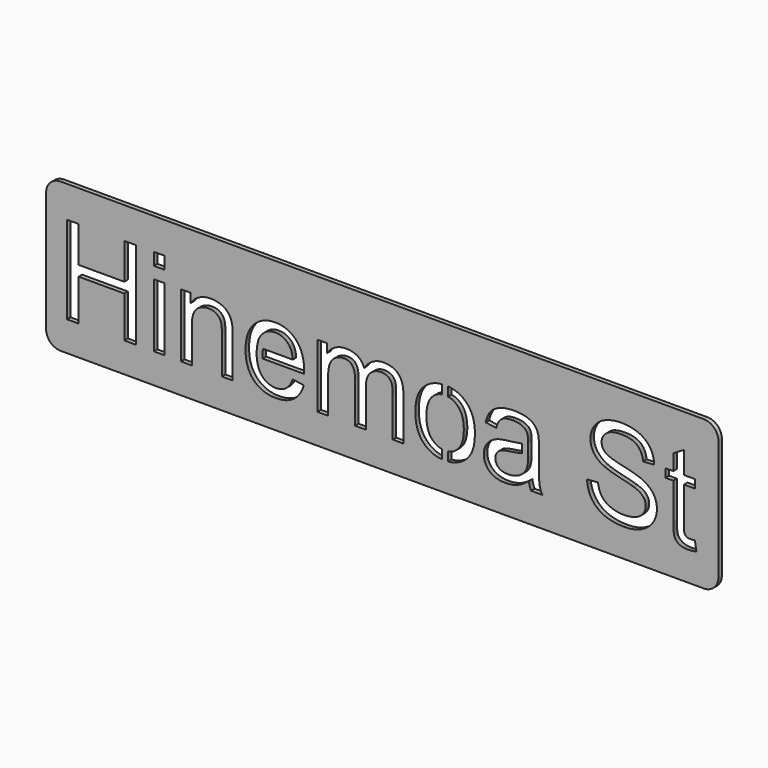
from build123d import *

# Parameters (mm, degrees)
F0_W     = 7.366985
F0_H     = 43.465211
F0_H_2   = 8.472033
F1_DEPTH = 3


# Not quite as in the source:
# - ends of sketch curves that miss each other by under 0.0002 mm in the source are joined


with BuildPart() as f1:
    # F0 (on Front) → F1 (new body)
    with BuildSketch(Plane.XZ):
        with BuildLine():
            Line((-230, 41), (-230, -41))
            ThreePointArc((-230, -41), (-227.0710678119, -48.0710678119), (-220, -51))
            Line((-220, -51), (220, -51))
            ThreePointArc((220, -51), (227.0710678119, -48.0710678119), (230, -41))
            Line((230, -41), (230, 41))
            ThreePointArc((230, 41), (227.0710678119, 48.0710678119), (220, 51))
            Line((220, 51), (-220, 51))
            ThreePointArc((-220, 51), (-227.0710678119, 48.0710678119), (-230, 41))
        make_face()
        Polygon((-207.702338, -2.27893), (-207.702338, -30.559967), (-215.64231, -30.559967), (-215.64231, 29.440033), (-207.702338, 29.440033), (-207.702338, 4.801561), (-176.515435, 4.801561), (-176.515435, 29.440033), (-168.575462, 29.440033), (-168.575462, -30.559967), (-176.515435, -30.559967), (-176.515435, -2.27893), align=None, mode=Mode.SUBTRACT)
        with Locations((-152.5727335, -8.8273615)):
            Rectangle(F0_W, F0_H, mode=Mode.SUBTRACT)
        Polygon((-130.308068, -6.821904), (-130.308068, -30.559967), (-137.675053, -30.559967), (-137.675053, 12.905244), (-131.044766, 12.905244), (-131.044766, 6.725163), (-130.429572, 7.592478), (-129.781124, 8.403837), (-129.099422, 9.159241), (-128.384466, 9.858689), (-127.636257, 10.502181), (-126.854793, 11.089717), (-126.040077, 11.621298), (-125.192106, 12.096922), (-124.310881, 12.516591), (-123.396403, 12.880304), (-122.448671, 13.188061), (-121.467686, 13.439862), (-120.453446, 13.635708), (-119.405953, 13.775597), (-118.325206, 13.859531), (-117.211205, 13.887509), (-116.238853, 13.865446), (-115.286325, 13.799259), (-114.353621, 13.688946), (-113.440742, 13.534508), (-112.547686, 13.335944), (-111.674456, 13.093256), (-110.821049, 12.806442), (-109.987467, 12.475504), (-109.189697, 12.108753), (-108.443726, 11.714504), (-107.749554, 11.292757), (-107.107181, 10.843512), (-106.516607, 10.366768), (-105.977832, 9.862526), (-105.490857, 9.330786), (-105.05568, 8.771547), (-104.661751, 8.18513), (-104.298518, 7.571854), (-103.96598, 6.931719), (-103.664139, 6.264726), (-103.392993, 5.570874), (-103.152542, 4.850163), (-102.942788, 4.102593), (-102.763729, 3.328164), (-102.714168, 3.060375), (-102.667805, 2.768606), (-102.624639, 2.452855), (-102.584671, 2.113123), (-102.5479, 1.74941), (-102.514326, 1.361716), (-102.48395, 0.950041), (-102.456772, 0.514385), (-102.432791, 0.054748), (-102.412007, -0.428871), (-102.394421, -0.93647), (-102.380032, -1.46805), (-102.368841, -2.023612), (-102.360847, -2.603154), (-102.356051, -3.206678), (-102.354452, -3.834183), (-102.354452, -30.559967), (-109.721437, -30.559967), (-109.721437, -4.120677), (-109.734867, -3.030657), (-109.775155, -2.011621), (-109.842302, -1.06357), (-109.936308, -0.186502), (-110.057172, 0.619582), (-110.204896, 1.354682), (-110.379478, 2.018797), (-110.580919, 2.611929), (-110.816573, 3.1555), (-111.093794, 3.670933), (-111.412582, 4.158229), (-111.772938, 4.617386), (-112.174861, 5.048406), (-112.618351, 5.451288), (-113.103408, 5.826032), (-113.630032, 6.172639), (-114.189271, 6.484393), (-114.772171, 6.754579), (-115.378732, 6.983199), (-116.008954, 7.170251), (-116.662838, 7.315736), (-117.340383, 7.419654), (-118.04159, 7.482005), (-118.766458, 7.502789), (-119.349757, 7.491118), (-119.922985, 7.456106), (-120.48614, 7.397752), (-121.039224, 7.316056), (-121.582235, 7.211019), (-122.115175, 7.08264), (-122.638042, 6.93092), (-123.150837, 6.755858), (-123.65356, 6.557455), (-124.146211, 6.33571), (-124.62879, 6.090623), (-125.101298, 5.822195), (-125.563732, 5.530426), (-126.016095, 5.215314), (-126.458386, 4.876861), (-126.890605, 4.515067), (-127.304438, 4.120658), (-127.691573, 3.684363), (-128.052008, 3.20618), (-128.385745, 2.686111), (-128.692783, 2.124154), (-128.973121, 1.520311), (-129.226761, 0.874581), (-129.453702, 0.186963), (-129.653944, -0.542541), (-129.827487, -1.313932), (-129.974331, -2.12721), (-130.094476, -2.982375), (-130.187922, -3.879427), (-130.25467, -4.818366), (-130.294718, -5.799192), align=None, mode=Mode.SUBTRACT)
        with BuildLine():
            ThreePointArc((-81.8910878389, -10.7100350654), (-81.9384658936, -7.6725767513), (-81.6083677497, -4.6527368704))
            Line((-81.6083677497, -4.6527368704), (-61.222119, -4.652737))
            Line((-61.222119, -4.652737), (-61.290545, -3.977909))
            Line((-61.290545, -3.977909), (-61.37304, -3.324505))
            Line((-61.37304, -3.324505), (-61.469604, -2.692524))
            Line((-61.469604, -2.692524), (-61.580237, -2.081966))
            Line((-61.580237, -2.081966), (-61.704938, -1.492831))
            Line((-61.704938, -1.492831), (-61.843709, -0.925119))
            Line((-61.843709, -0.925119), (-61.996548, -0.37883))
            Line((-61.996548, -0.37883), (-62.163456, 0.146036))
            Line((-62.163456, 0.146036), (-62.344434, 0.649478))
            Line((-62.344434, 0.649478), (-62.53948, 1.131498))
            Line((-62.53948, 1.131498), (-62.748595, 1.592094))
            Line((-62.748595, 1.592094), (-62.971778, 2.031268))
            Line((-62.971778, 2.031268), (-63.209031, 2.449018))
            Line((-63.209031, 2.449018), (-63.460353, 2.845345))
            Line((-63.460353, 2.845345), (-63.725743, 3.220249))
            Line((-63.725743, 3.220249), (-64.005203, 3.57373))
            Line((-64.005203, 3.57373), (-64.453329, 4.089163))
            Line((-64.453329, 4.089163), (-64.917762, 4.571343))
            Line((-64.917762, 4.571343), (-65.398503, 5.020268))
            Line((-65.398503, 5.020268), (-65.895551, 5.43594))
            Line((-65.895551, 5.43594), (-66.408905, 5.818358))
            Line((-66.408905, 5.818358), (-66.938567, 6.167523))
            Line((-66.938567, 6.167523), (-67.484536, 6.483433))
            Line((-67.484536, 6.483433), (-68.046813, 6.76609))
            Line((-68.046813, 6.76609), (-68.625396, 7.015493))
            Line((-68.625396, 7.015493), (-69.220286, 7.231643))
            Line((-69.220286, 7.231643), (-69.831484, 7.414538))
            Line((-69.831484, 7.414538), (-70.458989, 7.56418))
            Line((-70.458989, 7.56418), (-71.1028, 7.680568))
            Line((-71.1028, 7.680568), (-71.762919, 7.763703))
            Line((-71.762919, 7.763703), (-72.439345, 7.813583))
            Line((-72.439345, 7.813583), (-73.132079, 7.83021))
            Line((-73.132079, 7.83021), (-73.760143, 7.816941))
            Line((-73.760143, 7.816941), (-74.375577, 7.777132))
            Line((-74.375577, 7.777132), (-74.978381, 7.710785))
            Line((-74.978381, 7.710785), (-75.568555, 7.617898))
            Line((-75.568555, 7.617898), (-76.146099, 7.498472))
            Line((-76.146099, 7.498472), (-76.711014, 7.352507))
            Line((-76.711014, 7.352507), (-77.263298, 7.180003))
            Line((-77.263298, 7.180003), (-77.802952, 6.980961))
            Line((-77.802952, 6.980961), (-78.329976, 6.755379))
            Line((-78.329976, 6.755379), (-78.84437, 6.503258))
            Line((-78.84437, 6.503258), (-79.346134, 6.224598))
            Line((-79.346134, 6.224598), (-79.835267, 5.919399))
            Line((-79.835267, 5.919399), (-80.311771, 5.58766))
            Line((-80.311771, 5.58766), (-80.775645, 5.229383))
            Line((-80.775645, 5.229383), (-81.226889, 4.844567))
            Line((-81.226889, 4.844567), (-81.665503, 4.433212))
            Line((-81.665503, 4.433212), (-82.085731, 3.999634))
            Line((-82.085731, 3.999634), (-82.481818, 3.54815))
            Line((-82.481818, 3.54815), (-82.853765, 3.078761))
            Line((-82.853765, 3.078761), (-83.20157, 2.591465))
            Line((-83.20157, 2.591465), (-83.525235, 2.086264))
            Line((-83.525235, 2.086264), (-83.824758, 1.563157))
            Line((-83.824758, 1.563157), (-84.100141, 1.022144))
            Line((-84.100141, 1.022144), (-84.351383, 0.463225))
            Line((-84.351383, 0.463225), (-84.578484, -0.113599))
            Line((-84.578484, -0.113599), (-84.960261, -1.320966))
            ThreePointArc((-84.960261, -1.320966), (-85.8232752784, -5.9761863774), (-85.901515741, -10.7100800496))
            Line((-85.901515741, -10.7100800496), (-85.87971, -11.011642))
            ThreePointArc((-85.87971, -11.011642), (-85.6041419553, -13.325925097), (-85.1398797958, -15.6098481961))
            Line((-85.1398797958, -15.6098481961), (-84.68392, -17.033364))
            Line((-84.68392, -17.033364), (-84.41805, -17.705793))
            Line((-84.41805, -17.705793), (-84.12692, -18.352003))
            Line((-84.12692, -18.352003), (-83.81053, -18.971994))
            Line((-83.81053, -18.971994), (-83.468879, -19.565765))
            Line((-83.468879, -19.565765), (-83.101969, -20.133317))
            Line((-83.101969, -20.133317), (-82.709799, -20.67465))
            Line((-82.709799, -20.67465), (-82.292368, -21.189763))
            Line((-82.292368, -21.189763), (-81.849677, -21.678657))
            Line((-81.849677, -21.678657), (-81.387322, -22.139574))
            Line((-81.387322, -22.139574), (-80.910898, -22.570753))
            Line((-80.910898, -22.570753), (-80.420406, -22.972196))
            Line((-80.420406, -22.972196), (-79.915844, -23.343903))
            Line((-79.915844, -23.343903), (-79.397213, -23.685873))
            Line((-79.397213, -23.685873), (-78.864514, -23.998107))
            Line((-78.864514, -23.998107), (-78.317745, -24.280604))
            Line((-78.317745, -24.280604), (-77.756908, -24.533364))
            Line((-77.756908, -24.533364), (-77.182002, -24.756388))
            Line((-77.182002, -24.756388), (-76.593027, -24.949675))
            Line((-76.593027, -24.949675), (-75.989983, -25.113226))
            Line((-75.989983, -25.113226), (-75.37287, -25.247041))
            Line((-75.37287, -25.247041), (-74.741688, -25.351119))
            Line((-74.741688, -25.351119), (-74.096437, -25.42546))
            Line((-74.096437, -25.42546), (-73.437118, -25.470065))
            Line((-73.437118, -25.470065), (-72.763729, -25.484933))
            Line((-72.763729, -25.484933), (-71.769314, -25.451679))
            Line((-71.769314, -25.451679), (-70.81199, -25.351918))
            Line((-70.81199, -25.351918), (-69.891756, -25.185649))
            Line((-69.891756, -25.185649), (-69.008613, -24.952873))
            Line((-69.008613, -24.952873), (-68.162561, -24.653589))
            Line((-68.162561, -24.653589), (-67.3536, -24.287798))
            Line((-67.3536, -24.287798), (-66.581729, -23.855499))
            Line((-66.581729, -23.855499), (-65.846949, -23.356693))
            Line((-65.846949, -23.356693), (-65.14926, -22.784984))
            Line((-65.14926, -22.784984), (-64.488661, -22.133978))
            Line((-64.488661, -22.133978), (-63.865153, -21.403674))
            Line((-63.865153, -21.403674), (-63.278736, -20.594074))
            Line((-63.278736, -20.594074), (-62.72941, -19.705175))
            Line((-62.72941, -19.705175), (-62.217174, -18.736979))
            Line((-62.217174, -18.736979), (-61.742029, -17.689486))
            Line((-61.742029, -17.689486), (-61.303975, -16.562696))
            Line((-61.303975, -16.562696), (-53.691424, -17.504033))
            Line((-53.691424, -17.504033), (-53.928517, -18.326264))
            Line((-53.928517, -18.326264), (-54.18959, -19.125153))
            Line((-54.18959, -19.125153), (-54.474645, -19.900701))
            Line((-54.474645, -19.900701), (-54.783682, -20.652907))
            Line((-54.783682, -20.652907), (-55.116699, -21.381772))
            Line((-55.116699, -21.381772), (-55.473697, -22.087295))
            Line((-55.473697, -22.087295), (-55.854676, -22.769476))
            Line((-55.854676, -22.769476), (-56.259637, -23.428316))
            Line((-56.259637, -23.428316), (-56.688578, -24.063815))
            Line((-56.688578, -24.063815), (-57.1415, -24.675972))
            Line((-57.1415, -24.675972), (-57.618404, -25.264787))
            Line((-57.618404, -25.264787), (-58.119289, -25.83026))
            Line((-58.119289, -25.83026), (-58.644154, -26.372392))
            Line((-58.644154, -26.372392), (-59.193001, -26.891183))
            Line((-59.193001, -26.891183), (-59.765829, -27.386632))
            Line((-59.765829, -27.386632), (-60.362638, -27.858739))
            Line((-60.362638, -27.858739), (-60.981989, -28.304787))
            Line((-60.981989, -28.304787), (-61.622443, -28.722058))
            Line((-61.622443, -28.722058), (-62.284001, -29.110551))
            Line((-62.284001, -29.110551), (-62.966662, -29.470267))
            Line((-62.966662, -29.470267), (-63.670427, -29.801206))
            Line((-63.670427, -29.801206), (-64.395295, -30.103367))
            Line((-64.395295, -30.103367), (-65.141266, -30.376752))
            Line((-65.141266, -30.376752), (-65.90834, -30.621359))
            Line((-65.90834, -30.621359), (-66.696518, -30.837188))
            Line((-66.696518, -30.837188), (-67.5058, -31.024241))
            Line((-67.5058, -31.024241), (-68.336184, -31.182516))
            Line((-68.336184, -31.182516), (-69.187672, -31.312013))
            Line((-69.187672, -31.312013), (-70.060263, -31.412734))
            Line((-70.060263, -31.412734), (-70.953958, -31.484677))
            Line((-70.953958, -31.484677), (-71.868756, -31.527843))
            Line((-71.868756, -31.527843), (-72.804657, -31.542232))
            Line((-72.804657, -31.542232), (-73.981248, -31.51929))
            Line((-73.981248, -31.51929), (-75.126984, -31.450464))
            Line((-75.126984, -31.450464), (-76.241864, -31.335755))
            Line((-76.241864, -31.335755), (-77.325888, -31.175161))
            Line((-77.325888, -31.175161), (-78.379057, -30.968684))
            Line((-78.379057, -30.968684), (-79.40137, -30.716324))
            Line((-79.40137, -30.716324), (-80.392827, -30.418079))
            Line((-80.392827, -30.418079), (-81.353429, -30.073951))
            Line((-81.353429, -30.073951), (-82.283175, -29.683939))
            Line((-82.283175, -29.683939), (-83.182066, -29.248043))
            Line((-83.182066, -29.248043), (-84.050101, -28.766263))
            Line((-84.050101, -28.766263), (-84.88728, -28.238599))
            Line((-84.88728, -28.238599), (-85.693603, -27.665052))
            Line((-85.693603, -27.665052), (-86.469071, -27.045621))
            Line((-86.469071, -27.045621), (-87.213683, -26.380306))
            Line((-87.213683, -26.380306), (-87.92744, -25.669108))
            Line((-87.92744, -25.669108), (-88.603946, -24.916502))
            Line((-88.603946, -24.916502), (-89.236807, -24.126965))
            Line((-89.236807, -24.126965), (-89.826021, -23.300497))
            Line((-89.826021, -23.300497), (-90.371591, -22.437099))
            Line((-90.371591, -22.437099), (-90.873515, -21.536769))
            Line((-90.873515, -21.536769), (-91.331793, -20.599509))
            Line((-91.331793, -20.599509), (-91.746426, -19.625318))
            Line((-91.746426, -19.625318), (-92.117413, -18.614196))
            Line((-92.117413, -18.614196), (-92.444754, -17.566144))
            Line((-92.444754, -17.566144), (-92.72845, -16.48116))
            Line((-92.72845, -16.48116), (-92.968501, -15.359246))
            Line((-92.968501, -15.359246), (-93.164906, -14.2004))
            Line((-93.164906, -14.2004), (-93.317665, -13.004624))
            Line((-93.317665, -13.004624), (-93.426779, -11.771917))
            Line((-93.426779, -11.771917), (-93.492248, -10.502279))
            Line((-93.492248, -10.502279), (-93.51407, -9.195711))
            Line((-93.51407, -9.195711), (-93.492008, -7.843818))
            Line((-93.492008, -7.843818), (-93.42582, -6.530295))
            Line((-93.42582, -6.530295), (-93.315507, -5.255141))
            Line((-93.315507, -5.255141), (-93.161069, -4.018357))
            Line((-93.161069, -4.018357), (-92.962506, -2.819943))
            Line((-92.962506, -2.819943), (-92.719817, -1.659899))
            Line((-92.719817, -1.659899), (-92.433004, -0.538224))
            Line((-92.433004, -0.538224), (-92.102065, 0.545081))
            Line((-92.102065, 0.545081), (-91.727001, 1.590016))
            Line((-91.727001, 1.590016), (-91.307812, 2.596581))
            Line((-91.307812, 2.596581), (-90.844498, 3.564777))
            Line((-90.844498, 3.564777), (-90.337058, 4.494603))
            Line((-90.337058, 4.494603), (-89.785493, 5.38606))
            Line((-89.785493, 5.38606), (-89.189804, 6.239146))
            Line((-89.189804, 6.239146), (-88.549989, 7.053863))
            Line((-88.549989, 7.053863), (-87.866049, 7.83021))
            Line((-87.866049, 7.83021), (-87.146936, 8.563711))
            Line((-87.146936, 8.563711), (-86.401604, 9.24989))
            Line((-86.401604, 9.24989), (-85.630053, 9.888745))
            Line((-85.630053, 9.888745), (-84.832283, 10.480278))
            Line((-84.832283, 10.480278), (-84.008294, 11.024489))
            Line((-84.008294, 11.024489), (-83.158085, 11.521377))
            Line((-83.158085, 11.521377), (-82.281656, 11.970942))
            Line((-82.281656, 11.970942), (-81.379009, 12.373184))
            Line((-81.379009, 12.373184), (-80.450142, 12.728104))
            Line((-80.450142, 12.728104), (-79.495056, 13.035701))
            Line((-79.495056, 13.035701), (-78.513751, 13.295976))
            Line((-78.513751, 13.295976), (-77.506226, 13.508928))
            Line((-77.506226, 13.508928), (-76.472482, 13.674557))
            Line((-76.472482, 13.674557), (-75.412519, 13.792864))
            Line((-75.412519, 13.792864), (-74.326336, 13.863848))
            Line((-74.326336, 13.863848), (-73.213934, 13.887509))
            Line((-73.213934, 13.887509), (-72.136704, 13.864327))
            Line((-72.136704, 13.864327), (-71.084415, 13.794782))
            Line((-71.084415, 13.794782), (-70.057066, 13.678874))
            Line((-70.057066, 13.678874), (-69.054657, 13.516602))
            Line((-69.054657, 13.516602), (-68.077189, 13.307966))
            Line((-68.077189, 13.307966), (-67.12466, 13.052968))
            Line((-67.12466, 13.052968), (-66.197073, 12.751606))
            Line((-66.197073, 12.751606), (-65.294425, 12.40388))
            Line((-65.294425, 12.40388), (-64.416718, 12.009791))
            Line((-64.416718, 12.009791), (-63.563951, 11.569339))
            Line((-63.563951, 11.569339), (-62.736124, 11.082523))
            Line((-62.736124, 11.082523), (-61.933238, 10.549344))
            Line((-61.933238, 10.549344), (-61.155292, 9.969801))
            Line((-61.155292, 9.969801), (-60.402287, 9.343895))
            Line((-60.402287, 9.343895), (-59.674221, 8.671626))
            Line((-59.674221, 8.671626), (-58.971096, 7.952993))
            Line((-58.971096, 7.952993), (-58.302024, 7.192314))
            Line((-58.302024, 7.192314), (-57.676118, 6.393904))
            Line((-57.676118, 6.393904), (-57.093378, 5.557764))
            Line((-57.093378, 5.557764), (-56.553804, 4.683894))
            Line((-56.553804, 4.683894), (-56.057396, 3.772293))
            Line((-56.057396, 3.772293), (-55.604154, 2.822963))
            Line((-55.604154, 2.822963), (-55.194078, 1.835902))
            Line((-55.194078, 1.835902), (-54.827167, 0.811111))
            Line((-54.827167, 0.811111), (-54.503423, -0.251411))
            Line((-54.503423, -0.251411), (-54.222844, -1.351662))
            Line((-54.222844, -1.351662), (-53.985432, -2.489644))
            Line((-53.985432, -2.489644), (-53.791185, -3.665356))
            Line((-53.791185, -3.665356), (-53.640104, -4.878798))
            Line((-53.640104, -4.878798), (-53.532189, -6.12997))
            Line((-53.532189, -6.12997), (-53.467441, -7.418873))
            Line((-53.467441, -7.418873), (-53.445858, -8.745506))
            Line((-53.445858, -8.745506), (-53.448416, -9.113855))
            Line((-53.448416, -9.113855), (-53.456089, -9.56406))
            Line((-53.456089, -9.56406), (-53.468879, -10.09612))
            Line((-53.468879, -10.09612), (-53.486785, -10.710035))
            Line((-53.486785, -10.710035), (-81.8910878389, -10.7100350654))
        make_face(mode=Mode.SUBTRACT)
        Polygon((-37.07478, -8.008807), (-37.07478, -30.559967), (-44.441765, -30.559967), (-44.441765, 12.905244), (-37.852406, 12.905244), (-37.852406, 6.807018), (-37.319706, 7.585603), (-36.7448, 8.32518), (-36.127687, 9.025747), (-35.468368, 9.687304), (-34.766842, 10.309853), (-34.023109, 10.893392), (-33.237169, 11.437923), (-32.409023, 11.943444), (-31.545065, 12.399084), (-30.65169, 12.793972), (-29.728898, 13.128108), (-28.77669, 13.401493), (-27.795065, 13.614125), (-26.784023, 13.766005), (-25.743564, 13.857133), (-24.673688, 13.887509), (-23.4935, 13.856174), (-22.367669, 13.762168), (-21.296194, 13.605492), (-20.279077, 13.386145), (-19.316317, 13.104127), (-18.407914, 12.759439), (-17.553868, 12.352081), (-16.75418, 11.882052), (-16.010127, 11.355747), (-15.322989, 10.779562), (-14.692767, 10.153496), (-14.119459, 9.47755), (-13.603067, 8.751723), (-13.143589, 7.976015), (-12.741027, 7.150427), (-12.39538, 6.274958), (-11.738618, 7.19679), (-11.057556, 8.05915), (-10.352193, 8.862036), (-9.622529, 9.605449), (-8.868564, 10.289389), (-8.090298, 10.913856), (-7.287732, 11.47885), (-6.460864, 11.984371), (-5.609696, 12.430419), (-4.734227, 12.816994), (-3.834457, 13.144096), (-2.910387, 13.411725), (-1.962015, 13.61988), (-0.989343, 13.768563), (0.00763, 13.857773), (1.028904, 13.887509), (1.825555, 13.87352), (2.598864, 13.831553), (3.348833, 13.761608), (4.075459, 13.663686), (4.778744, 13.537785), (5.458687, 13.383907), (6.115289, 13.20205), (6.748549, 12.992216), (7.358468, 12.754403), (7.945045, 12.488613), (8.50828, 12.194845), (9.048174, 11.873099), (9.564726, 11.523375), (10.057937, 11.145673), (10.527806, 10.739993), (10.974333, 10.306336), (11.395601, 9.843581), (11.78969, 9.35061), (12.1566, 8.827423), (12.496332, 8.27402), (12.808885, 7.690401), (13.09426, 7.076565), (13.352456, 6.432514), (13.583474, 5.758246), (13.787313, 5.053762), (13.963974, 4.319062), (14.113456, 3.554146), (14.235759, 2.759013), (14.330884, 1.933665), (14.39883, 1.0781), (14.439598, 0.192319), (14.453187, -0.723678), (14.453187, -30.559967), (7.12713, -30.559967), (7.12713, -3.17934), (7.115939, -2.112981), (7.082366, -1.124002), (7.02641, -0.212401), (6.948072, 0.62182), (6.847351, 1.378663), (6.724248, 2.058126), (6.578763, 2.660211), (6.410896, 3.184917), (6.213611, 3.659103), (5.979876, 4.109627), (5.709689, 4.53649), (5.403051, 4.939692), (5.059962, 5.319232), (4.680421, 5.675111), (4.26443, 6.007329), (3.811987, 6.315886), (3.331087, 6.594066), (2.829722, 6.835156), (2.307894, 7.039155), (1.765602, 7.206063), (1.202846, 7.33588), (0.619627, 7.428607), (0.015943, 7.484243), (-0.608204, 7.502789), (-1.175117, 7.490878), (-1.729879, 7.455146), (-2.27249, 7.395593), (-2.802952, 7.312219), (-3.321263, 7.205024), (-3.827423, 7.074007), (-4.321433, 6.919169), (-4.803293, 6.74051), (-5.273002, 6.53803), (-5.730561, 6.311729), (-6.175969, 6.061606), (-6.609227, 5.787663), (-7.030335, 5.489898), (-7.439292, 5.168311), (-7.836099, 4.822904), (-8.220755, 4.453675), (-8.587506, 4.058228), (-8.930595, 3.634162), (-9.250023, 3.18148), (-9.545789, 2.70018), (-9.817895, 2.190262), (-10.066338, 1.651727), (-10.291121, 1.084575), (-10.492242, 0.488805), (-10.669702, -0.135582), (-10.823501, -0.788587), (-10.953638, -1.470209), (-11.060114, -2.180448), (-11.142929, -2.919305), (-11.202082, -3.686779), (-11.237574, -4.482871), (-11.249405, -5.30758), (-11.249405, -30.559967), (-18.61639, -30.559967), (-18.61639, -2.319858), (-18.644527, -1.130397), (-18.728941, -0.017675), (-18.86963, 1.018307), (-19.066594, 1.97755), (-19.319834, 2.860053), (-19.62935, 3.665817), (-19.995141, 4.394842), (-20.417208, 5.047127), (-20.651263, 5.344492), (-20.903225, 5.622673), (-21.173092, 5.881668), (-21.460864, 6.121479), (-21.766543, 6.342105), (-22.090128, 6.543546), (-22.431618, 6.725802), (-22.791014, 6.888873), (-23.168317, 7.03276), (-23.563525, 7.157461), (-23.976639, 7.262978), (-24.407658, 7.34931), (-24.856584, 7.416457), (-25.323416, 7.464419), (-25.808153, 7.493196), (-26.310796, 7.502789), (-27.081068, 7.477209), (-27.836632, 7.400469), (-28.577487, 7.27257), (-29.303634, 7.093512), (-30.015072, 6.863293), (-30.711802, 6.581916), (-31.393824, 6.249378), (-32.061137, 5.865681), (-32.698394, 5.432743), (-33.290247, 4.952482), (-33.836696, 4.424898), (-34.33774, 3.849992), (-34.793381, 3.227763), (-35.203617, 2.558212), (-35.568449, 1.841337), (-35.887877, 1.077141), (-36.166057, 0.245797), (-36.407147, -0.672518), (-36.611146, -1.677805), (-36.778054, -2.770063), (-36.907872, -3.949292), (-37.000598, -5.215492), (-37.056234, -6.568664), align=None, mode=Mode.SUBTRACT)
        Polygon((22.726657, -11.499172), (22.660709, -10.183411), (22.638726, -8.827361), (22.664946, -7.342613), (22.743604, -5.906787), (22.8747, -4.519881), (23.058235, -3.181898), (23.294209, -1.892835), (23.582621, -0.652694), (23.923472, 0.538526), (24.316762, 1.680824), (24.76249, 2.774201), (25.260657, 3.818657), (25.811262, 4.814191), (26.414306, 5.760804), (27.069789, 6.658495), (27.77771, 7.507265), (28.53807, 8.307114), (29.350868, 9.058041), (30.061347, 9.642859), (30.791011, 10.189948), (31.53986, 10.699306), (32.307894, 11.170933), (33.095113, 11.604831), (33.901516, 12.000998), (34.727105, 12.359435), (35.571878, 12.680142), (36.435836, 12.963119), (37.318979, 13.208365), (38.221307, 13.415881), (39.142819, 13.585667), (40.083517, 13.717723), (41.020718, 13.80982), (41.020718, 7.644671), (41.014941, 7.643957), (40.375766, 7.530926), (39.751299, 7.385601), (39.14154, 7.207981), (38.54649, 6.998067), (37.966148, 6.755858), (37.400514, 6.481355), (36.849589, 6.174557), (36.313373, 5.835465), (35.791864, 5.464078), (35.285064, 5.060397), (34.792973, 4.624421), (34.315589, 4.15615), (33.852915, 3.655585), (33.411823, 3.122406), (32.999189, 2.556293), (32.615012, 1.957246), (32.259293, 1.325265), (31.932031, 0.66035), (31.633227, -0.037499), (31.36288, -0.768283), (31.120991, -1.532), (30.907559, -2.328651), (30.722586, -3.158236), (30.566069, -4.020755), (30.43801, -4.916209), (30.338409, -5.844596), (30.267265, -6.805917), (30.224579, -7.800172), (30.21035, -8.827361), (30.224579, -9.854631), (30.267265, -10.849126), (30.338409, -11.810846), (30.43801, -12.739793), (30.566069, -13.635966), (30.722586, -14.499364), (30.907559, -15.329989), (31.120991, -16.127839), (31.36288, -16.892915), (31.633227, -17.625217), (31.932031, -18.324745), (32.259293, -18.991498), (32.615012, -19.625478), (32.999189, -20.226683), (33.411823, -20.795115), (33.852915, -21.330772), (34.315589, -21.833815), (34.792973, -22.304403), (35.285064, -22.742538), (35.791864, -23.148217), (36.313373, -23.521443), (36.849589, -23.862214), (37.400514, -24.17053), (37.966148, -24.446393), (38.54649, -24.689801), (39.14154, -24.900754), (39.751299, -25.079253), (40.375766, -25.225298), (41.014941, -25.338888), (41.020718, -25.339605), (41.020718, -31.464942), (40.793676, -31.450784), (39.721163, -31.336474), (38.675988, -31.17644), (37.658151, -30.970683), (36.667653, -30.719201), (35.704493, -30.421996), (34.768672, -30.079067), (33.860189, -29.690413), (32.979044, -29.256036), (32.125238, -28.775935), (31.298771, -28.25011), (30.499641, -27.678561), (29.727851, -27.061289), (28.983398, -26.398292), (28.266284, -25.689571), (27.584822, -24.937845), (26.947325, -24.14583), (26.353794, -23.313527), (25.804228, -22.440936), (25.298627, -21.528056), (24.836991, -20.574889), (24.419321, -19.581433), (24.045616, -18.547689), (23.715876, -17.473657), (23.430102, -16.359336), (23.188293, -15.204727), (22.990449, -14.009831), (22.83657, -12.774646), align=None, mode=Mode.SUBTRACT)
        Polygon((45.020718, -31.447252), (45.020718, -25.336707), (45.647765, -25.224019), (46.268555, -25.077255), (46.874956, -24.897876), (47.466969, -24.685884), (48.044593, -24.441277), (48.607828, -24.164056), (49.156675, -23.85422), (49.691133, -23.51177), (50.211202, -23.136707), (50.716883, -22.729028), (51.208176, -22.288736), (51.685079, -21.815829), (52.147594, -21.310308), (52.588686, -20.771374), (53.00132, -20.198226), (53.385497, -19.590865), (53.741216, -18.949292), (54.068478, -18.273505), (54.367282, -17.563506), (54.637629, -16.819293), (54.879518, -16.040867), (55.092949, -15.228229), (55.277923, -14.381377), (55.43444, -13.500313), (55.562499, -12.585035), (55.6621, -11.635545), (55.733244, -10.651841), (55.77593, -9.633925), (55.790159, -8.581795), (55.77585, -7.589219), (55.732924, -6.627178), (55.66138, -5.695673), (55.56122, -4.794704), (55.432441, -3.924272), (55.275045, -3.084374), (55.089032, -2.275013), (54.874402, -1.496188), (54.631154, -0.747899), (54.359288, -0.030145), (54.058805, 0.657072), (53.729705, 1.313754), (53.371988, 1.9399), (52.985653, 2.53551), (52.5707, 3.100584), (52.12713, 3.635122), (51.662297, 4.138165), (51.183555, 4.608753), (50.690904, 5.046887), (50.184344, 5.452567), (49.663875, 5.825792), (49.129496, 6.166563), (48.581209, 6.47488), (48.019013, 6.750742), (47.442908, 6.99415), (46.852893, 7.205104), (46.24897, 7.383603), (45.631138, 7.529648), (45.020718, 7.639405), (45.020718, 13.807804), (45.21035, 13.795741), (46.266796, 13.681032), (47.297662, 13.520439), (48.302949, 13.313962), (49.282655, 13.061601), (50.236782, 12.763356), (51.165329, 12.419228), (52.068297, 12.029216), (52.945684, 11.59332), (53.797492, 11.11154), (54.62372, 10.583877), (55.424368, 10.010329), (56.199436, 9.390898), (56.948924, 8.725584), (57.672833, 8.014385), (58.361729, 7.262738), (59.00618, 6.476079), (59.606187, 5.654408), (60.161748, 4.797724), (60.672865, 3.906028), (61.139536, 2.979319), (61.561763, 2.017598), (61.939545, 1.020865), (62.272882, -0.010881), (62.561774, -1.077638), (62.806221, -2.179409), (63.006223, -3.316192), (63.16178, -4.487987), (63.272892, -5.694794), (63.33956, -6.936614), (63.361782, -8.213446), (63.35195, -9.248229), (63.322453, -10.255034), (63.273292, -11.233862), (63.204466, -12.184711), (63.115976, -13.107583), (63.007822, -14.002476), (62.880003, -14.869392), (62.732519, -15.70833), (62.565371, -16.51929), (62.378558, -17.302272), (62.172081, -18.057276), (61.94594, -18.784302), (61.700134, -19.48335), (61.434663, -20.154421), (61.149529, -20.797513), (60.844729, -21.412627), (60.521145, -22.00536), (60.179654, -22.581305), (59.820258, -23.140464), (59.442956, -23.682835), (59.047748, -24.208421), (58.634634, -24.717219), (58.203614, -25.209231), (57.754688, -25.684455), (57.287857, -26.142894), (56.803119, -26.584545), (56.300476, -27.00941), (55.779927, -27.417488), (55.241472, -27.808779), (54.685111, -28.183283), (54.110844, -28.541001), (53.518672, -28.881932), (52.302672, -29.505439), (51.059173, -30.045813), (49.788176, -30.503052), (48.489681, -30.877157), (47.163688, -31.168127), (45.810196, -31.375963), align=None, mode=Mode.SUBTRACT)
        Polygon((95.754524, -4.058125), (95.748057, -10.012906), (95.469239, -10.083969), (94.73286, -10.259831), (93.965146, -10.431855), (93.166097, -10.600042), (92.335712, -10.764392), (91.473992, -10.924906), (90.580937, -11.081582), (89.656547, -11.234421), (88.700821, -11.383424), (87.71376, -11.528589), (86.619584, -11.694858), (85.608542, -11.866243), (84.680635, -12.042743), (83.835861, -12.22436), (83.074223, -12.411093), (82.395718, -12.602941), (81.800348, -12.799906), (81.288112, -13.001986), (80.830873, -13.218455), (80.400493, -13.458586), (79.996972, -13.722378), (79.620309, -14.009831), (79.270505, -14.320945), (78.94756, -14.655721), (78.651474, -15.014158), (78.382246, -15.396256), (78.142435, -15.795621), (77.934599, -16.205857), (77.758738, -16.626965), (77.614852, -17.058944), (77.50294, -17.501794), (77.423003, -17.955516), (77.375041, -18.420109), (77.359054, -18.895574), (77.393906, -19.616925), (77.498464, -20.30758), (77.672726, -20.967539), (77.916694, -21.596802), (78.230366, -22.19537), (78.613743, -22.763241), (79.066826, -23.300417), (79.589613, -23.806898), (80.179547, -24.267334), (80.834071, -24.666379), (81.553183, -25.004033), (82.336885, -25.280295), (83.185175, -25.495165), (84.098054, -25.648644), (85.075523, -25.740731), (86.11758, -25.771427), (87.166992, -25.74233), (88.186987, -25.655039), (89.177565, -25.509554), (90.138726, -25.305874), (91.070471, -25.044001), (91.972799, -24.723934), (92.84571, -24.345672), (93.689204, -23.909217), (94.490491, -23.422241), (95.236782, -22.892419), (95.928077, -22.319751), (96.564374, -21.704237), (97.145676, -21.045877), (97.67198, -20.34467), (98.143288, -19.600618), (98.559599, -18.813719), (98.83778, -18.152481), (99.07887, -17.417061), (99.282869, -16.60746), (99.449777, -15.723678), (99.579594, -14.765714), (99.672321, -13.733569), (99.727957, -12.627242), (99.746503, -11.446734), (99.756095, -2.613386), (99.764408, -2.286604), (99.771443, -1.994355), (99.777198, -1.736638), (99.781675, -1.513454), (99.784872, -1.324803), (99.786791, -1.170685), (99.78743, -1.051099), (99.779277, -0.498735), (99.754816, 0.032845), (99.714048, 0.543642), (99.656973, 1.033655), (99.583591, 1.502885), (99.493902, 1.951331), (99.387906, 2.378993), (99.265602, 2.785872), (99.126992, 3.171967), (98.972074, 3.537279), (98.800849, 3.881807), (98.613317, 4.205551), (98.409478, 4.508512), (98.189332, 4.790689), (97.952878, 5.052083), (97.700118, 5.292693), (97.336405, 5.595015), (96.951269, 5.877831), (96.54471, 6.141144), (96.116728, 6.384951), (95.667322, 6.609254), (95.196494, 6.814052), (94.704243, 6.999346), (94.190568, 7.165135), (93.65547, 7.31142), (93.09895, 7.4382), (92.521006, 7.545475), (91.921639, 7.633246), (91.300849, 7.701512), (90.658636, 7.750273), (89.995, 7.77953), (89.309941, 7.789283), (88.670845, 7.782168), (88.053013, 7.760825), (87.456444, 7.725253), (86.881138, 7.675452), (86.327095, 7.611423), (85.794316, 7.533165), (85.282799, 7.440678), (84.792546, 7.333962), (84.323556, 7.213017), (83.87583, 7.077844), (83.449366, 6.928442), (83.044166, 6.764811), (82.660229, 6.586952), (82.297556, 6.394863), (81.956145, 6.188546), (81.635998, 5.968), (81.331518, 5.729389), (81.037111, 5.468874), (80.752775, 5.186457), (80.478511, 4.882137), (80.21432, 4.555915), (79.960201, 4.20779), (79.716153, 3.837762), (79.482178, 3.445831), (79.258275, 3.031998), (79.044443, 2.596262), (78.840684, 2.138623), (78.646997, 1.659081), (78.463382, 1.157637), (78.289839, 0.63429), (78.126368, 0.089041), (77.972969, -0.478112), (70.769695, 0.504153), (71.035086, 1.632542), (71.340125, 2.705296), (71.684813, 3.722413), (72.069149, 4.683894), (72.493135, 5.589739), (72.956769, 6.439948), (73.460051, 7.23452), (74.002983, 7.973457), (74.597074, 8.664112), (75.253836, 9.313839), (75.973268, 9.922639), (76.75537, 10.49051), (77.600143, 11.017454), (78.507587, 11.503471), (79.477701, 11.94856), (80.510486, 12.35272), (81.59571, 12.712437), (82.72314, 13.02419), (83.892777, 13.287982), (85.10462, 13.503812), (86.35867, 13.671679), (87.654927, 13.791585), (88.99339, 13.863528), (90.374061, 13.887509), (91.732988, 13.867045), (93.026687, 13.805654), (94.255157, 13.703334), (95.418399, 13.560087), (96.516412, 13.375913), (97.549197, 13.150811), (98.516753, 12.884781), (99.419081, 12.577823), (100.260017, 12.23985), (101.043399, 11.880773), (101.769226, 11.500593), (102.437499, 11.09931), (103.048216, 10.676923), (103.60138, 10.233433), (104.096989, 9.76884), (104.535043, 9.283143), (104.928972, 8.770588), (105.292205, 8.225418), (105.624743, 7.647634), (105.926584, 7.037236), (106.19773, 6.394224), (106.438181, 5.718597), (106.647935, 5.010356), (106.826994, 4.269501), (106.913326, 3.75151), (106.988147, 3.138873), (107.051457, 2.431592), (107.103256, 1.629665), (107.143544, 0.733092), (107.172321, -0.258125), (107.189588, -1.343988), (107.195343, -2.524496), (107.195343, -12.347143), (107.197182, -13.601753), (107.202697, -14.797369), (107.21189, -15.933992), (107.22476, -17.011621), (107.241307, -18.030257), (107.261531, -18.9899), (107.285432, -19.890549), (107.31301, -20.732204), (107.344265, -21.514867), (107.379198, -22.238535), (107.417807, -22.903211), (107.460094, -23.508893), (107.506058, -24.055581), (107.555699, -24.543276), (107.609016, -24.971978), (107.666011, -25.341686), (107.798067, -26.018592), (107.9589, -26.688463), (108.148511, -27.3513), (108.366898, -28.007102), (108.614063, -28.65587), (108.890005, -29.297604), (109.194725, -29.932303), (109.528222, -30.559967), (101.833815, -30.559967), (101.560111, -29.974829), (101.311987, -29.36539), (101.089443, -28.73165), (100.892478, -28.07361), (100.721093, -27.391268), (100.575288, -26.684626), (100.455063, -25.953683), (100.360418, -25.198439), (99.342022, -26.036178), (98.333218, -26.809967), (97.334007, -27.519807), (96.344388, -28.165697), (95.364362, -28.747638), (94.393928, -29.265629), (93.433086, -29.71967), (92.481837, -30.109762), (91.526751, -30.445497), (90.554398, -30.736468), (89.564779, -30.982673), (88.557894, -31.184114), (87.533743, -31.340791), (86.492325, -31.452702), (85.43364, -31.519849), (84.35769, -31.542232), (83.475346, -31.528563), (82.618902, -31.487555), (81.788358, -31.419209), (80.983713, -31.323524), (80.204967, -31.200501), (79.452122, -31.05014), (78.725175, -30.87244), (78.024129, -30.667402), (77.348982, -30.435026), (76.699734, -30.175311), (76.076386, -29.888257), (75.478938, -29.573865), (74.907389, -29.232135), (74.36174, -28.863067), (73.84199, -28.466659), (73.34814, -28.042914), (72.882267, -27.597905), (72.446451, -27.137708), (72.040692, -26.662324), (71.664988, -26.171751), (71.319341, -25.66599), (71.00375, -25.145041), (70.718216, -24.608904), (70.462737, -24.05758), (70.237315, -23.491067), (70.041949, -22.909366), (69.87664, -22.312477), (69.741387, -21.7004), (69.63619, -21.073135), (69.561049, -20.430682), (69.515965, -19.773042), (69.500936, -19.100213), (69.523639, -18.310756), (69.591745, -17.538565), (69.705255, -16.783641), (69.86417, -16.045983), (70.068488, -15.325592), (70.318211, -14.622467), (70.613338, -13.936608), (70.95387, -13.268016), (71.331172, -12.624364), (71.736612, -12.013327), (72.17019, -11.434903), (72.631905, -10.889094), (73.121758, -10.375899), (73.63975, -9.895318), (74.185878, -9.447352), (74.760145, -9.032), (75.357753, -8.645105), (75.973907, -8.282511), (76.608606, -7.944218), (77.261851, -7.630226), (77.93364, -7.340535), (78.623975, -7.075144), (79.332856, -6.834055), (80.060282, -6.617266), (80.637106, -6.474658), (81.282996, -6.33333), (81.997952, -6.193281), (82.781973, -6.05451), (83.63506, -5.917019), (84.557212, -5.780806), (85.54843, -5.645873), (86.608713, -5.512218), (87.705607, -5.377604), (88.76573, -5.239793), (89.789082, -5.098784), (90.775664, -4.954578), (91.725474, -4.807175), (92.638513, -4.656574), (93.514782, -4.502775), (94.354279, -4.345779), (95.157005, -4.185585), align=None, mode=Mode.SUBTRACT)
        Polygon((140.229428, -12.767611), (140.174192, -12.030193), (140.142137, -11.283023), (147.631905, -10.62818), (147.786983, -11.728431), (147.986185, -12.778163), (148.229513, -13.777374), (148.516966, -14.726065), (148.848545, -15.624236), (149.224248, -16.471887), (149.644077, -17.269018), (150.108031, -18.015629), (150.62762, -18.719713), (151.214357, -19.389264), (151.868241, -20.024283), (152.589272, -20.624769), (153.37745, -21.190723), (154.232775, -21.722143), (155.155247, -22.219031), (156.144866, -22.681386), (157.184045, -23.098657), (158.2552, -23.460291), (159.358329, -23.76629), (160.493433, -24.016652), (161.660512, -24.211378), (162.859565, -24.350468), (164.090594, -24.433923), (165.353597, -24.461741), (166.472713, -24.440637), (167.558576, -24.377327), (168.611185, -24.271811), (169.630541, -24.124087), (170.616642, -23.934157), (171.56949, -23.70202), (172.489084, -23.427677), (173.375425, -23.111127), (174.21732, -22.757806), (175.00358, -22.373149), (175.734203, -21.957158), (176.40919, -21.509831), (177.028541, -21.031168), (177.592256, -20.521171), (178.100335, -19.979838), (178.552778, -19.40717), (178.950864, -18.81212), (179.295872, -18.20364), (179.587801, -17.581731), (179.826653, -16.946393), (180.012426, -16.297625), (180.145121, -15.635428), (180.224738, -14.959801), (180.251278, -14.270745), (180.225698, -13.575933), (180.148958, -12.903504), (180.021059, -12.253457), (179.842001, -11.625792), (179.611782, -11.02051), (179.330404, -10.43761), (178.997867, -9.877093), (178.61417, -9.338958), (178.171639, -8.822565), (177.662601, -8.327276), (177.087055, -7.85309), (176.445002, -7.400008), (175.736441, -6.968029), (174.961373, -6.557153), (174.119797, -6.167381), (173.211714, -5.798712), (172.88701, -5.676968), (172.516583, -5.547071), (172.100431, -5.40902), (171.638556, -5.262815), (171.130956, -5.108457), (170.577633, -4.945945), (169.978586, -4.77528), (169.333815, -4.596461), (168.64332, -4.409489), (167.907101, -4.214363), (167.125158, -4.011083), (166.297492, -3.79965), (165.424101, -3.580063), (164.504987, -3.352323), (163.540148, -3.116429), (162.529586, -2.872382), (161.515506, -2.625137), (160.540116, -2.379651), (159.603416, -2.135923), (158.705404, -1.893954), (157.846083, -1.653744), (157.02545, -1.415292), (156.243508, -1.178599), (155.500254, -0.943664), (154.79569, -0.710488), (154.129816, -0.479071), (153.502631, -0.249412), (152.914136, -0.021512), (152.36433, 0.204629), (151.853213, 0.429012), (151.380786, 0.651637), (150.947048, 0.872502), (149.906909, 1.452205), (148.935196, 2.0658), (148.031909, 2.713289), (147.197048, 3.394671), (146.430613, 4.109947), (145.732604, 4.859115), (145.103021, 5.642177), (144.541864, 6.459133), (144.047854, 7.305504), (143.619712, 8.176817), (143.257438, 9.073069), (142.961032, 9.994262), (142.730494, 10.940395), (142.565824, 11.911469), (142.467022, 12.907483), (142.434088, 13.928437), (142.474376, 15.054908), (142.595241, 16.162833), (142.796682, 17.252213), (143.078699, 18.323048), (143.441293, 19.375337), (143.884463, 20.409081), (144.40821, 21.42428), (145.012533, 22.420933), (145.694235, 23.378577), (146.450118, 24.276748), (147.280183, 25.115446), (148.184429, 25.894671), (149.162857, 26.614423), (150.215466, 27.274702), (151.342256, 27.875508), (152.543228, 28.416841), (153.798558, 28.896462), (155.088419, 29.312134), (156.412814, 29.663856), (157.771741, 29.951629), (159.165201, 30.175452), (160.593194, 30.335326), (162.05572, 30.431251), (163.552778, 30.463225), (165.195961, 30.429652), (166.789903, 30.328931), (168.334604, 30.161064), (169.830063, 29.926049), (171.276282, 29.623888), (172.673259, 29.254579), (174.020995, 28.818124), (175.31949, 28.314521), (175.947235, 28.03802), (176.556594, 27.74569), (177.147567, 27.437534), (177.720155, 27.113549), (178.274358, 26.773738), (178.810175, 26.418098), (179.327607, 26.046631), (179.826653, 25.659337), (180.307313, 25.256215), (180.769588, 24.837266), (181.213478, 24.402489), (181.638982, 23.951885), (182.046101, 23.485453), (182.434834, 23.003194), (182.805182, 22.505107), (183.157144, 21.991193), (183.803034, 20.93027), (184.369627, 19.834815), (184.856922, 18.704827), (185.26492, 17.540306), (185.593621, 16.341252), (185.843024, 15.107666), (186.01313, 13.839547), (186.103938, 12.536895), (178.491387, 11.963907), (178.403216, 12.664155), (178.292184, 13.342659), (178.15829, 13.999421), (178.001533, 14.634439), (177.821915, 15.247715), (177.619435, 15.839248), (177.394093, 16.409039), (177.145889, 16.957086), (176.874823, 17.483391), (176.580895, 17.987952), (176.264105, 18.470771), (175.924453, 18.931847), (175.561939, 19.371181), (175.176563, 19.788771), (174.768325, 20.184619), (174.337226, 20.558723), (173.881505, 20.910605), (173.399406, 21.239786), (172.890927, 21.546264), (172.356069, 21.83004), (171.794832, 22.091114), (171.207216, 22.329486), (170.593221, 22.545155), (169.952846, 22.738123), (169.286093, 22.908389), (168.59296, 23.055952), (167.873448, 23.180814), (167.127557, 23.282973), (166.355286, 23.36243), (165.556636, 23.419185), (164.731608, 23.453238), (163.8802, 23.46459), (162.995058, 23.454278), (162.140453, 23.423342), (161.316383, 23.371783), (160.52285, 23.2996), (159.759852, 23.206793), (159.02739, 23.093363), (158.325464, 22.959308), (157.654074, 22.80463), (157.01322, 22.629329), (156.402902, 22.433403), (155.823119, 22.216854), (155.273873, 21.979682), (154.755162, 21.721885), (154.266988, 21.443465), (153.809349, 21.144421), (153.382246, 20.824753), (152.983281, 20.490537), (152.610056, 20.147848), (152.26257, 19.796685), (151.940824, 19.437049), (151.644818, 19.068939), (151.374551, 18.692356), (151.130024, 18.3073), (150.911237, 17.913771), (150.718189, 17.511768), (150.550881, 17.101292), (150.409313, 16.682343), (150.293484, 16.25492), (150.203395, 15.819024), (150.139046, 15.374655), (150.100437, 14.921813), (150.087567, 14.460497), (150.124018, 13.670081), (150.233372, 12.915476), (150.415628, 12.196684), (150.670786, 11.513703), (150.998847, 10.866534), (151.399811, 10.255176), (151.873677, 9.67963), (152.420445, 9.139896), (152.735796, 8.878583), (153.108862, 8.61647), (153.539642, 8.353557), (154.028136, 8.089845), (154.574345, 7.825334), (155.178268, 7.560024), (155.839906, 7.293914), (156.559258, 7.027004), (157.336325, 6.759296), (158.171106, 6.490788), (159.063602, 6.22148), (160.013812, 5.951373), (161.021736, 5.680467), (162.087375, 5.408762), (163.210728, 5.136257), (164.391796, 4.862952), (165.57798, 4.591407), (166.716681, 4.324178), (167.807899, 4.061265), (168.851636, 3.802669), (169.847889, 3.54839), (170.79666, 3.298427), (171.697949, 3.052781), (172.551755, 2.811452), (173.358079, 2.574439), (174.11692, 2.341742), (174.828278, 2.113363), (175.492154, 1.8893), (176.108548, 1.669553), (176.677458, 1.454123), (177.198887, 1.24301), (177.672833, 1.036213), (178.939673, 0.412385), (180.12082, -0.25173), (181.216276, -0.956134), (182.226039, -1.700827), (183.150109, -2.485807), (183.988488, -3.311076), (184.741173, -4.176632), (185.408167, -5.082477), (185.993305, -6.026053), (186.500425, -7.0048), (186.929526, -8.01872), (187.280609, -9.067812), (187.553673, -10.152076), (187.74872, -11.271512), (187.865747, -12.426121), (187.904756, -13.615902), (187.86191, -14.804403), (187.733372, -15.975639), (187.519141, -17.129608), (187.219217, -18.266311), (186.833602, -19.385747), (186.362294, -20.487917), (185.805294, -21.572821), (185.162601, -22.640458), (184.439652, -23.670046), (183.641881, -24.640799), (182.76929, -25.552719), (181.821878, -26.405806), (180.799645, -27.200059), (179.702591, -27.935479), (178.530716, -28.612065), (177.28402, -29.229817), (175.979769, -29.781382), (174.63523, -30.259404), (173.250404, -30.663885), (171.825288, -30.994824), (170.359885, -31.252221), (168.854194, -31.436076), (167.308214, -31.546388), (165.721946, -31.583159), (164.714181, -31.573887), (163.727041, -31.546069), (162.760524, -31.499705), (161.81463, -31.434797), (160.889361, -31.351342), (159.984715, -31.249343), (159.100692, -31.128798), (158.237294, -30.989708), (157.394519, -30.832072), (156.572368, -30.655891), (155.770841, -30.461165), (154.989937, -30.247893), (154.229657, -30.016076), (153.490001, -29.765714), (152.770969, -29.496806), (152.07256, -29.209353), (151.393736, -28.903275), (150.733457, -28.578491), (150.091723, -28.235002), (149.468535, -27.872808), (148.863893, -27.491909), (148.277795, -27.092304), (147.710243, -26.673994), (147.161237, -26.236979), (146.630775, -25.781259), (146.118859, -25.306834), (145.625489, -24.813703), (145.150664, -24.301867), (144.694384, -23.771326), (144.256649, -23.222079), (143.83746, -22.654127), (143.436816, -22.06747), (143.057036, -21.466585), (142.700438, -20.855947), (142.367021, -20.235556), (142.056786, -19.605414), (141.769732, -18.965519), (141.505861, -18.315872), (141.265171, -17.656472), (141.047662, -16.98732), (140.853336, -16.308416), (140.682191, -15.61976), (140.534228, -14.921351), (140.409446, -14.21319), (140.307846, -13.495277), align=None, mode=Mode.SUBTRACT)
        Polygon((212.939715, -24.095949), (213.404628, -24.037755), (213.893842, -23.970608), (214.957962, -30.478112), (214.190568, -30.631591), (213.443638, -30.764606), (212.717171, -30.877157), (212.011168, -30.969244), (211.32563, -31.040867), (210.660554, -31.092027), (210.015943, -31.122723), (209.391796, -31.132955), (208.417205, -31.11313), (207.49889, -31.053657), (206.636851, -30.954536), (205.831087, -30.815765), (205.081598, -30.637346), (204.388385, -30.419278), (203.751448, -30.161562), (203.170786, -29.864196), (202.638726, -29.534536), (202.147594, -29.179936), (201.697389, -28.800396), (201.288112, -28.395915), (200.919763, -27.966494), (200.592342, -27.512133), (200.305848, -27.032831), (200.060282, -26.528589), (199.951248, -26.252407), (199.849248, -25.940573), (199.754283, -25.593088), (199.666353, -25.20995), (199.585456, -24.791161), (199.511595, -24.336719), (199.444767, -23.846626), (199.384975, -23.320881), (199.332216, -22.759484), (199.286492, -22.162436), (199.247803, -21.529735), (199.216148, -20.861383), (199.191527, -20.157378), (199.173941, -19.417722), (199.16339, -18.642414), (199.159872, -17.831454), (199.159872, 7.175367), (193.757417, 7.175367), (193.757417, 12.905244), (199.159872, 12.905244), (199.159872, 23.669228), (206.48593, 28.089419), (206.48593, 12.905244), (213.893842, 12.905244), (213.893842, 7.175367), (206.48593, 7.175367), (206.48593, -18.240731), (206.492005, -18.993417), (206.51023, -19.675758), (206.540606, -20.287755), (206.583133, -20.829408), (206.63781, -21.300716), (206.704637, -21.701679), (206.783615, -22.032298), (206.874743, -22.292573), (207.099845, -22.719756), (207.386339, -23.100895), (207.734224, -23.43599), (208.143501, -23.725042), (208.375318, -23.849744), (208.630797, -23.957818), (208.909936, -24.049266), (209.212737, -24.124087), (209.5392, -24.182281), (209.889323, -24.223848), (210.263108, -24.248789), (210.660554, -24.257102), (210.979663, -24.252626), (211.323072, -24.239196), (211.690781, -24.216814), (212.082792, -24.185479), (212.499103, -24.14519), align=None, mode=Mode.SUBTRACT)
        with Locations((-152.5727335, 25.2040165)):
            Rectangle(F0_W, F0_H_2, mode=Mode.SUBTRACT)
    extrude(amount=F1_DEPTH)


solid = f1.part
